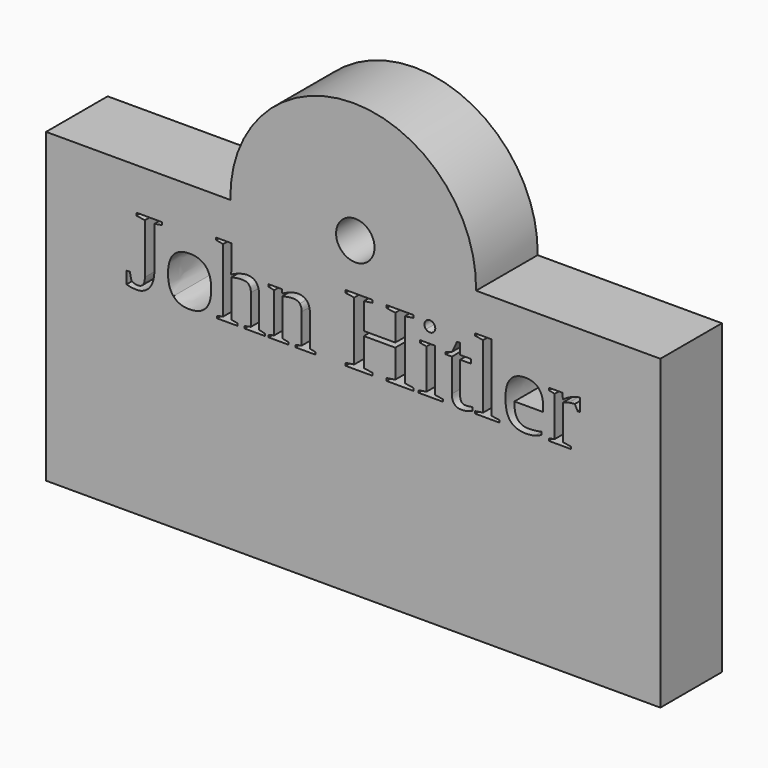
from build123d import *

# Parameters (mm, degrees)
F0_R     = 2.5
F1_DEPTH = 10


with BuildPart() as f1:
    # F0 (on Front) → F1 (new body)
    with BuildSketch(Plane.XZ):
        with BuildLine():
            Line((-40.177900088, 40.0071958417), (-40.177900088, 0.1012184115))
            Line((-40.177900088, 0.1012184115), (39.6340547723, 0.1012184115))
            Line((39.6340547723, 0.1012184115), (39.6340547723, 40.0071958417))
            Line((39.6340547723, 40.0071958417), (15.6904683142, 40.0071958417))
            ThreePointArc((15.6904683142, 40.0071958417), (-0.2719226578, 56.2958275849), (-16.2343136299, 40.0071958417))
            Line((-16.2343136299, 40.0071958417), (-40.177900088, 40.0071958417))
        make_face()
        with BuildLine():
            Line((-27.3462693782, 27.556749315), (-27.3462693782, 34.0698867662))
            Line((-27.3462693782, 34.0698867662), (-28.4587231986, 34.2376870631))
            Line((-28.4587231986, 34.2376870631), (-28.4587231986, 34.5815740914))
            Line((-28.4587231986, 34.5815740914), (-25.1192901288, 34.5815740914))
            Line((-25.1192901288, 34.5815740914), (-25.1192901288, 34.2376870631))
            Line((-25.1192901288, 34.2376870631), (-26.1033042157, 34.0698867662))
            Line((-26.1033042157, 34.0698867662), (-26.1033042157, 28.6961340472))
            add(Edge.make_bspline(
                [(-26.1033042157, 28.6961340472), (-26.1033042157, 27.8281300421), (-26.368470117, 27.1776449404)],
                knots=[0, 0, 0, 1, 1, 1], degree=2))
            add(Edge.make_bspline(
                [(-26.368470117, 27.1776449404), (-26.6336360184, 26.5271598388), (-27.174325864, 26.1480554642)],
                knots=[0, 0, 0, 1, 1, 1], degree=2))
            add(Edge.make_bspline(
                [(-27.174325864, 26.1480554642), (-27.7150157097, 25.7689510897), (-28.3820736802, 25.7689510897)],
                knots=[0, 0, 0, 1, 1, 1], degree=2))
            add(Edge.make_bspline(
                [(-28.3820736802, 25.7689510897), (-29.2107171218, 25.7689510897), (-29.7224044471, 25.9636822984)],
                knots=[0, 0, 0, 1, 1, 1], degree=2))
            Line((-29.7224044471, 25.9636822984), (-29.7224044471, 27.5443196634))
            Line((-29.7224044471, 27.5443196634), (-29.293581466, 27.5443196634))
            Line((-29.293581466, 27.5443196634), (-29.1009218658, 26.6431699206))
            add(Edge.make_bspline(
                [(-29.1009218658, 26.6431699206), (-28.9766253496, 26.4960857097), (-28.7497842074, 26.4111497569)],
                knots=[0, 0, 0, 1, 1, 1], degree=2))
            add(Edge.make_bspline(
                [(-28.7497842074, 26.4111497569), (-28.5229430653, 26.3262138042), (-28.2515623382, 26.3262138042)],
                knots=[0, 0, 0, 1, 1, 1], degree=2))
            add(Edge.make_bspline(
                [(-28.2515623382, 26.3262138042), (-27.3462693782, 26.3262138042), (-27.3462693782, 27.556749315)],
                knots=[0, 0, 0, 1, 1, 1], degree=2))
        make_face(mode=Mode.SUBTRACT)
        with BuildLine():
            add(Edge.make_bspline(
                [(-19.4213306633, 31.3477930605), (-18.7159479336, 30.5481521393), (-18.7159479336, 28.9737296002)],
                knots=[0, 0, 0, 1, 1, 1], degree=2))
            add(Edge.make_bspline(
                [(-18.7159479336, 28.9737296002), (-18.7159479336, 25.7689510897), (-21.5644097642, 25.7689510897)],
                knots=[0, 0, 0, 1, 1, 1], degree=2))
            add(Edge.make_bspline(
                [(-21.5644097642, 25.7689510897), (-22.9358146601, 25.7689510897), (-23.634982564, 26.5913797055)],
                knots=[0, 0, 0, 1, 1, 1], degree=2))
            add(Edge.make_bspline(
                [(-23.634982564, 26.5913797055), (-24.3341504678, 27.4138083213), (-24.3341504678, 28.9737296002)],
                knots=[0, 0, 0, 1, 1, 1], degree=2))
            add(Edge.make_bspline(
                [(-24.3341504678, 28.9737296002), (-24.3341504678, 30.5150064016), (-23.634982564, 31.3312201916)],
                knots=[0, 0, 0, 1, 1, 1], degree=2))
            add(Edge.make_bspline(
                [(-23.634982564, 31.3312201916), (-22.9358146601, 32.1474339816), (-21.5126195491, 32.1474339816)],
                knots=[0, 0, 0, 1, 1, 1], degree=2))
            add(Edge.make_bspline(
                [(-21.5126195491, 32.1474339816), (-20.1267133929, 32.1474339816), (-19.4213306633, 31.3477930605)],
                knots=[0, 0, 0, 1, 1, 1], degree=2))
        make_face(mode=Mode.SUBTRACT)
        with BuildLine():
            Line((-16.0995062666, 35.0994762424), (-16.0995062666, 32.4643900981))
            add(Edge.make_bspline(
                [(-16.0995062666, 32.4643900981), (-16.0995062666, 31.7911173017), (-16.1450816559, 31.4928056627)],
                knots=[0, 0, 0, 1, 1, 1], degree=2))
            add(Edge.make_bspline(
                [(-16.1450816559, 31.4928056627), (-15.67896972, 31.7579715641), (-15.0864896592, 31.9527027728)],
                knots=[0, 0, 0, 1, 1, 1], degree=2))
            add(Edge.make_bspline(
                [(-15.0864896592, 31.9527027728), (-14.4940095985, 32.1474339816), (-14.0859027034, 32.1474339816)],
                knots=[0, 0, 0, 1, 1, 1], degree=2))
            add(Edge.make_bspline(
                [(-14.0859027034, 32.1474339816), (-13.2966198253, 32.1474339816), (-12.8957635604, 31.6875368715)],
                knots=[0, 0, 0, 1, 1, 1], degree=2))
            add(Edge.make_bspline(
                [(-12.8957635604, 31.6875368715), (-12.4949072955, 31.2276397614), (-12.4949072955, 30.3534209305)],
                knots=[0, 0, 0, 1, 1, 1], degree=2))
            Line((-12.4949072955, 30.3534209305), (-12.4949072955, 26.353144716))
            Line((-12.4949072955, 26.353144716), (-11.7553430239, 26.1915592449))
            Line((-11.7553430239, 26.1915592449), (-11.7553430239, 25.8994624317))
            Line((-11.7553430239, 25.8994624317), (-14.3779995166, 25.8994624317))
            Line((-14.3779995166, 25.8994624317), (-14.3779995166, 26.1915592449))
            Line((-14.3779995166, 26.1915592449), (-13.5680005524, 26.353144716))
            Line((-13.5680005524, 26.353144716), (-13.5680005524, 30.2767714121))
            add(Edge.make_bspline(
                [(-13.5680005524, 30.2767714121), (-13.5680005524, 31.3892252325), (-14.6431654179, 31.3892252325)],
                knots=[0, 0, 0, 1, 1, 1], degree=2))
            add(Edge.make_bspline(
                [(-14.6431654179, 31.3892252325), (-15.2522183475, 31.3892252325), (-16.0995062666, 31.2007088496)],
                knots=[0, 0, 0, 1, 1, 1], degree=2))
            Line((-16.0995062666, 31.2007088496), (-16.0995062666, 26.353144716))
            Line((-16.0995062666, 26.353144716), (-15.2770776508, 26.1915592449))
            Line((-15.2770776508, 26.1915592449), (-15.2770776508, 25.8994624317))
            Line((-15.2770776508, 25.8994624317), (-17.9453095329, 25.8994624317))
            Line((-17.9453095329, 25.8994624317), (-17.9453095329, 26.1915592449))
            Line((-17.9453095329, 26.1915592449), (-17.1746711321, 26.353144716))
            Line((-17.1746711321, 26.353144716), (-17.1746711321, 34.652008784))
            Line((-17.1746711321, 34.652008784), (-18.0799640921, 34.8073794293))
            Line((-18.0799640921, 34.8073794293), (-18.0799640921, 35.0994762424))
            Line((-18.0799640921, 35.0994762424), (-16.0995062666, 35.0994762424))
        make_face(mode=Mode.SUBTRACT)
        with BuildLine():
            Line((-9.5428650347, 31.9858485105), (-9.4827883852, 31.4928056627))
            add(Edge.make_bspline(
                [(-9.4827883852, 31.4928056627), (-8.9856023202, 31.7786876501), (-8.4221247799, 31.9630608159)],
                knots=[0, 0, 0, 1, 1, 1], degree=2))
            add(Edge.make_bspline(
                [(-8.4221247799, 31.9630608159), (-7.8586472396, 32.1474339816), (-7.4836860822, 32.1474339816)],
                knots=[0, 0, 0, 1, 1, 1], degree=2))
            add(Edge.make_bspline(
                [(-7.4836860822, 32.1474339816), (-6.6944032041, 32.1474339816), (-6.2925111349, 31.6875368715)],
                knots=[0, 0, 0, 1, 1, 1], degree=2))
            add(Edge.make_bspline(
                [(-6.2925111349, 31.6875368715), (-5.8906190657, 31.2276397614), (-5.8906190657, 30.3534209305)],
                knots=[0, 0, 0, 1, 1, 1], degree=2))
            Line((-5.8906190657, 30.3534209305), (-5.8906190657, 26.353144716))
            Line((-5.8906190657, 26.353144716), (-5.1531264027, 26.1915592449))
            Line((-5.1531264027, 26.1915592449), (-5.1531264027, 25.8994624317))
            Line((-5.1531264027, 25.8994624317), (-7.7737112868, 25.8994624317))
            Line((-7.7737112868, 25.8994624317), (-7.7737112868, 26.1915592449))
            Line((-7.7737112868, 26.1915592449), (-6.9657839312, 26.353144716))
            Line((-6.9657839312, 26.353144716), (-6.9657839312, 30.2374108487))
            add(Edge.make_bspline(
                [(-6.9657839312, 30.2374108487), (-6.9657839312, 30.7739574771), (-7.2278424196, 31.0815913548)],
                knots=[0, 0, 0, 1, 1, 1], degree=2))
            add(Edge.make_bspline(
                [(-7.2278424196, 31.0815913548), (-7.4899009081, 31.3892252325), (-8.0409487967, 31.3892252325)],
                knots=[0, 0, 0, 1, 1, 1], degree=2))
            add(Edge.make_bspline(
                [(-8.0409487967, 31.3892252325), (-8.6230708145, 31.3892252325), (-9.4703587336, 31.2007088496)],
                knots=[0, 0, 0, 1, 1, 1], degree=2))
            Line((-9.4703587336, 31.2007088496), (-9.4703587336, 26.353144716))
            Line((-9.4703587336, 26.353144716), (-8.6479301177, 26.1915592449))
            Line((-8.6479301177, 26.1915592449), (-8.6479301177, 25.8994624317))
            Line((-8.6479301177, 25.8994624317), (-11.2768014363, 25.8994624317))
            Line((-11.2768014363, 25.8994624317), (-11.2768014363, 26.1915592449))
            Line((-11.2768014363, 26.1915592449), (-10.5455235991, 26.353144716))
            Line((-10.5455235991, 26.353144716), (-10.5455235991, 31.5321662262))
            Line((-10.5455235991, 31.5321662262), (-11.2768014363, 31.6937516973))
            Line((-11.2768014363, 31.6937516973), (-11.2768014363, 31.9858485105))
            Line((-11.2768014363, 31.9858485105), (-9.5428650347, 31.9858485105))
        make_face(mode=Mode.SUBTRACT)
        Polygon((2.2218002279, 25.8994624317), (-1.2564306184, 25.8994624317), (-1.2564306184, 26.24334946), (-0.1419051894, 26.4173645827), (-0.1419051894, 34.0698867662), (-1.2564306184, 34.2376870631), (-1.2564306184, 34.5815740914), (2.2218002279, 34.5815740914), (2.2218002279, 34.2376870631), (1.1072747989, 34.0698867662), (1.1072747989, 30.6579473953), (5.1924869661, 30.6579473953), (5.1924869661, 34.0698867662), (4.0779615371, 34.2376870631), (4.0779615371, 34.5815740914), (7.547905949, 34.5815740914), (7.547905949, 34.2376870631), (6.4354521286, 34.0698867662), (6.4354521286, 26.4173645827), (7.547905949, 26.24334946), (7.547905949, 25.8994624317), (4.0779615371, 25.8994624317), (4.0779615371, 26.24334946), (5.1924869661, 26.4173645827), (5.1924869661, 30.0758253775), (1.1072747989, 30.0758253775), (1.1072747989, 26.4173645827), (2.2218002279, 26.24334946), align=None, mode=Mode.SUBTRACT)
        with BuildLine():
            add(Edge.make_bspline(
                [(10.1829920934, 34.4717788354), (10.3901529538, 34.264617975), (10.3901529538, 33.9725211618)],
                knots=[0, 0, 0, 1, 1, 1], degree=2))
            add(Edge.make_bspline(
                [(10.3901529538, 33.9725211618), (10.3901529538, 33.6866391745), (10.1829920934, 33.4794783141)],
                knots=[0, 0, 0, 1, 1, 1], degree=2))
            add(Edge.make_bspline(
                [(10.1829920934, 33.4794783141), (9.975831233, 33.2723174536), (9.6858060284, 33.2723174536)],
                knots=[0, 0, 0, 1, 1, 1], degree=2))
            add(Edge.make_bspline(
                [(9.6858060284, 33.2723174536), (9.399924041, 33.2723174536), (9.1927631806, 33.4794783141)],
                knots=[0, 0, 0, 1, 1, 1], degree=2))
            add(Edge.make_bspline(
                [(9.1927631806, 33.4794783141), (8.9856023202, 33.6866391745), (8.9856023202, 33.9725211618)],
                knots=[0, 0, 0, 1, 1, 1], degree=2))
            add(Edge.make_bspline(
                [(8.9856023202, 33.9725211618), (8.9856023202, 34.264617975), (9.1927631806, 34.4717788354)],
                knots=[0, 0, 0, 1, 1, 1], degree=2))
            add(Edge.make_bspline(
                [(9.1927631806, 34.4717788354), (9.399924041, 34.6789396958), (9.6858060284, 34.6789396958)],
                knots=[0, 0, 0, 1, 1, 1], degree=2))
            add(Edge.make_bspline(
                [(9.6858060284, 34.6789396958), (9.975831233, 34.6789396958), (10.1829920934, 34.4717788354)],
                knots=[0, 0, 0, 1, 1, 1], degree=2))
        make_face(mode=Mode.SUBTRACT)
        Polygon((10.325933087, 31.9858485105), (10.325933087, 26.353144716), (11.3679522149, 26.1915592449), (11.3679522149, 25.8994624317), (8.2149639195, 25.8994624317), (8.2149639195, 26.1915592449), (9.2507682215, 26.353144716), (9.2507682215, 31.5321662262), (8.3910506508, 31.6937516973), (8.3910506508, 31.9858485105), align=None, mode=Mode.SUBTRACT)
        with BuildLine():
            add(Edge.make_bspline(
                [(14.5727307254, 25.869424107), (14.145979353, 25.7689510897), (13.7834478473, 25.7689510897)],
                knots=[0, 0, 0, 1, 1, 1], degree=2))
            add(Edge.make_bspline(
                [(13.7834478473, 25.7689510897), (13.161965266, 25.7689510897), (12.8543313883, 26.1387332255)],
                knots=[0, 0, 0, 1, 1, 1], degree=2))
            add(Edge.make_bspline(
                [(12.8543313883, 26.1387332255), (12.5466975106, 26.5085153613), (12.5466975106, 27.1755733318)],
                knots=[0, 0, 0, 1, 1, 1], degree=2))
            Line((12.5466975106, 27.1755733318), (12.5466975106, 31.4410154476))
            Line((12.5466975106, 31.4410154476), (11.7511998066, 31.4410154476))
            Line((11.7511998066, 31.4410154476), (11.7511998066, 31.7331122608))
            Line((11.7511998066, 31.7331122608), (12.5591271622, 31.9858485105))
            Line((12.5591271622, 31.9858485105), (13.2137554811, 33.3634682322))
            Line((13.2137554811, 33.3634682322), (13.6218623761, 33.3634682322))
            Line((13.6218623761, 33.3634682322), (13.6218623761, 31.9858485105))
            Line((13.6218623761, 31.9858485105), (15.0139833581, 31.9858485105))
            Line((15.0139833581, 31.9858485105), (15.0139833581, 31.4410154476))
            Line((15.0139833581, 31.4410154476), (13.6218623761, 31.4410154476))
            Line((13.6218623761, 31.4410154476), (13.6218623761, 27.2915834137))
            add(Edge.make_bspline(
                [(13.6218623761, 27.2915834137), (13.6218623761, 26.871046867), (13.8124503677, 26.6576711808)],
                knots=[0, 0, 0, 1, 1, 1], degree=2))
            add(Edge.make_bspline(
                [(13.8124503677, 26.6576711808), (14.0030383593, 26.4442954946), (14.3137796499, 26.4442954946)],
                knots=[0, 0, 0, 1, 1, 1], degree=2))
            add(Edge.make_bspline(
                [(14.3137796499, 26.4442954946), (14.6887408072, 26.4442954946), (15.2273590443, 26.5478759248)],
                knots=[0, 0, 0, 1, 1, 1], degree=2))
            Line((15.2273590443, 26.5478759248), (15.2273590443, 26.1252677696))
            add(Edge.make_bspline(
                [(15.2273590443, 26.1252677696), (14.9994820978, 25.9698971243), (14.5727307254, 25.869424107)],
                knots=[0, 0, 0, 1, 1, 1], degree=2))
        make_face(mode=Mode.SUBTRACT)
        Polygon((17.6801436315, 35.0994762424), (17.6801436315, 26.353144716), (18.7221627594, 26.1915592449), (18.7221627594, 25.8994624317), (15.569174464, 25.8994624317), (15.569174464, 26.1915592449), (16.604978766, 26.353144716), (16.604978766, 34.652008784), (15.569174464, 34.8073794293), (15.569174464, 35.0994762424), align=None, mode=Mode.SUBTRACT)
        with Locations((0, 40.6422099371)):
            Circle(F0_R, mode=Mode.SUBTRACT)
        with BuildLine():
            Line((24.4128715948, 28.9612999485), (20.6715464558, 28.9612999485))
            Line((20.6715464558, 28.9612999485), (20.6715464558, 28.8452898667))
            add(Edge.make_bspline(
                [(20.6715464558, 28.8452898667), (20.6715464558, 27.9524265584), (20.8683492732, 27.457312102)],
                knots=[0, 0, 0, 1, 1, 1], degree=2))
            add(Edge.make_bspline(
                [(20.8683492732, 27.457312102), (21.0651520906, 26.9621976456), (21.4763663985, 26.7032465701)],
                knots=[0, 0, 0, 1, 1, 1], degree=2))
            add(Edge.make_bspline(
                [(21.4763663985, 26.7032465701), (21.8875807064, 26.4442954946), (22.5546386769, 26.4442954946)],
                knots=[0, 0, 0, 1, 1, 1], degree=2))
            add(Edge.make_bspline(
                [(22.5546386769, 26.4442954946), (22.904740531, 26.4442954946), (23.3832821186, 26.5023005355)],
                knots=[0, 0, 0, 1, 1, 1], degree=2))
            add(Edge.make_bspline(
                [(23.3832821186, 26.5023005355), (23.8618237061, 26.5603055764), (24.1725649967, 26.630740269)],
                knots=[0, 0, 0, 1, 1, 1], degree=2))
            Line((24.1725649967, 26.630740269), (24.1725649967, 26.2682087632))
            add(Edge.make_bspline(
                [(24.1725649967, 26.2682087632), (23.8618237061, 26.0672627286), (23.3283844906, 25.9181069092)],
                knots=[0, 0, 0, 1, 1, 1], degree=2))
            add(Edge.make_bspline(
                [(23.3283844906, 25.9181069092), (22.794945275, 25.7689510897), (22.2376825605, 25.7689510897)],
                knots=[0, 0, 0, 1, 1, 1], degree=2))
            add(Edge.make_bspline(
                [(22.2376825605, 25.7689510897), (20.8186306667, 25.7689510897), (20.1619307392, 26.5333746646)],
                knots=[0, 0, 0, 1, 1, 1], degree=2))
            add(Edge.make_bspline(
                [(20.1619307392, 26.5333746646), (19.5052308117, 27.2977982395), (19.5052308117, 28.9882308604)],
                knots=[0, 0, 0, 1, 1, 1], degree=2))
            add(Edge.make_bspline(
                [(19.5052308117, 28.9882308604), (19.5052308117, 30.5792262683), (20.1722887822, 31.363330125)],
                knots=[0, 0, 0, 1, 1, 1], degree=2))
            add(Edge.make_bspline(
                [(20.1722887822, 31.363330125), (20.8393467528, 32.1474339816), (22.0760970894, 32.1474339816)],
                knots=[0, 0, 0, 1, 1, 1], degree=2))
            add(Edge.make_bspline(
                [(22.0760970894, 32.1474339816), (24.4128715948, 32.1474339816), (24.4128715948, 29.4916317512)],
                knots=[0, 0, 0, 1, 1, 1], degree=2))
            Line((24.4128715948, 29.4916317512), (24.4128715948, 28.9612999485))
        make_face(mode=Mode.SUBTRACT)
        with BuildLine():
            Line((29.073990954, 32.1474339816), (29.1713565584, 32.1474339816))
            Line((29.1713565584, 32.1474339816), (29.1713565584, 30.50257675))
            Line((29.1713565584, 30.50257675), (28.8937610054, 30.50257675))
            Line((28.8937610054, 30.50257675), (28.5167282395, 31.2152101098))
            add(Edge.make_bspline(
                [(28.5167282395, 31.2152101098), (28.1935572972, 31.2152101098), (27.750233056, 31.1271667441)],
                knots=[0, 0, 0, 1, 1, 1], degree=2))
            add(Edge.make_bspline(
                [(27.750233056, 31.1271667441), (27.3069088147, 31.0391233784), (26.9837378725, 30.8982539934)],
                knots=[0, 0, 0, 1, 1, 1], degree=2))
            Line((26.9837378725, 30.8982539934), (26.9837378725, 26.353144716))
            Line((26.9837378725, 26.353144716), (28.0257570003, 26.1915592449))
            Line((28.0257570003, 26.1915592449), (28.0257570003, 25.8994624317))
            Line((28.0257570003, 25.8994624317), (25.1379346062, 25.8994624317))
            Line((25.1379346062, 25.8994624317), (25.1379346062, 26.1915592449))
            Line((25.1379346062, 26.1915592449), (25.9085730069, 26.353144716))
            Line((25.9085730069, 26.353144716), (25.9085730069, 31.5321662262))
            Line((25.9085730069, 31.5321662262), (25.1379346062, 31.6937516973))
            Line((25.1379346062, 31.6937516973), (25.1379346062, 31.9858485105))
            Line((25.1379346062, 31.9858485105), (26.9112315713, 31.9858485105))
            Line((26.9112315713, 31.9858485105), (26.9713082208, 31.2276397614))
            add(Edge.make_bspline(
                [(26.9713082208, 31.2276397614), (27.3586990298, 31.5508107037), (28.0226495874, 31.8491223426)],
                knots=[0, 0, 0, 1, 1, 1], degree=2))
            add(Edge.make_bspline(
                [(28.0226495874, 31.8491223426), (28.686600145, 32.1474339816), (29.073990954, 32.1474339816)],
                knots=[0, 0, 0, 1, 1, 1], degree=2))
        make_face(mode=Mode.SUBTRACT)
    extrude(amount=F1_DEPTH)


solid = f1.part
